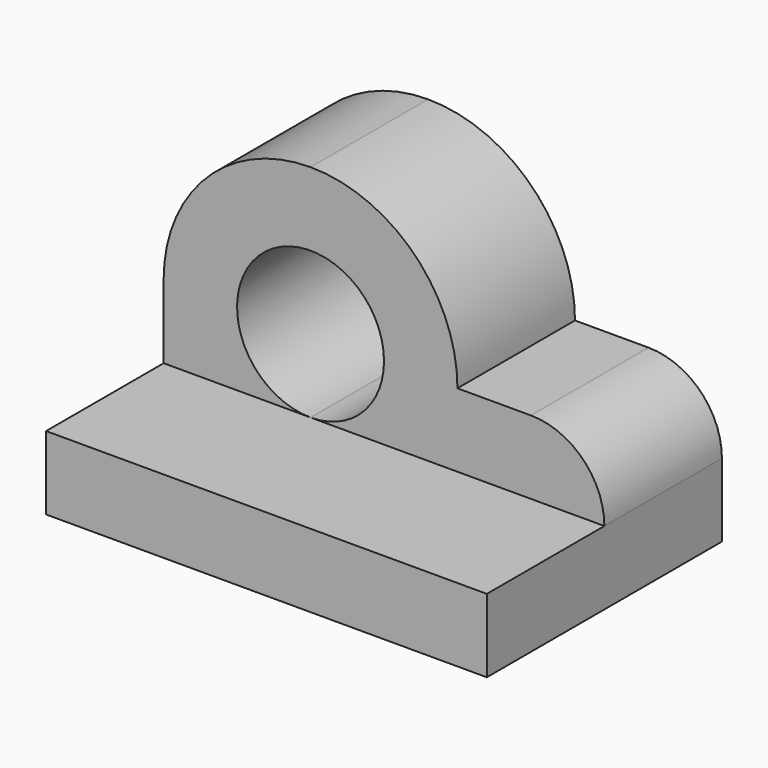
from build123d import *

# Parameters (mm, degrees)
F0_W     = 60
F0_H     = 10
F1_DEPTH = 40
F2_W     = 20
F2_H     = 20
F3_DEPTH = 10
F4_W     = 40
F4_H     = 20
F5_DEPTH = 30
F6_R     = 10
F7_R     = 19.99999
F9_DEPTH = 25


# Not quite as in the source:
# - a fillet or chamfer is up to 0.001 mm smaller than in the source, because OpenCascade refuses the exact size


with BuildPart() as f1:
    # F0 (on Front) → F1 (new body)
    with BuildSketch(Plane.XZ):
        with Locations((30, 5)):
            Rectangle(F0_W, F0_H)
    extrude(amount=F1_DEPTH)

    # F2 (on face) → F3 (join)
    with BuildSketch(Plane.XY.offset(10)):
        with Locations((50, -10)):
            Rectangle(F2_W, F2_H)
    extrude(amount=F3_DEPTH)

    # F4 (on face) → F5 (join)
    with BuildSketch(Plane.XY.offset(10)):
        with Locations((20, -10)):
            Rectangle(F4_W, F4_H)
    extrude(amount=F5_DEPTH)

    # F6
    f6_edges = [f1.edges().sort_by_distance(p)[0] for p in [
        (60, -10, 20),
    ]]
    fillet(f6_edges, radius=F6_R)

    # F7 (radius 20 in the source; OpenCascade refuses exactly that, so slightly less here)
    f7_edges = [f1.edges().sort_by_distance(p)[0] for p in [
        (40, -10, 40),
        (0, -10, 40),
    ]]
    fillet(f7_edges, radius=F7_R)

    # F8 (on face) → F9 (cut)
    with BuildSketch(Plane.XZ.offset(20)):
        with BuildLine():
            ThreePointArc((20, 10), (27.0710678119, 12.9289321881), (30, 20))
            ThreePointArc((30, 20), (12.9289321881, 27.0710678119), (20, 10))
        make_face()
    extrude(amount=-F9_DEPTH, mode=Mode.SUBTRACT)


solid = f1.part
